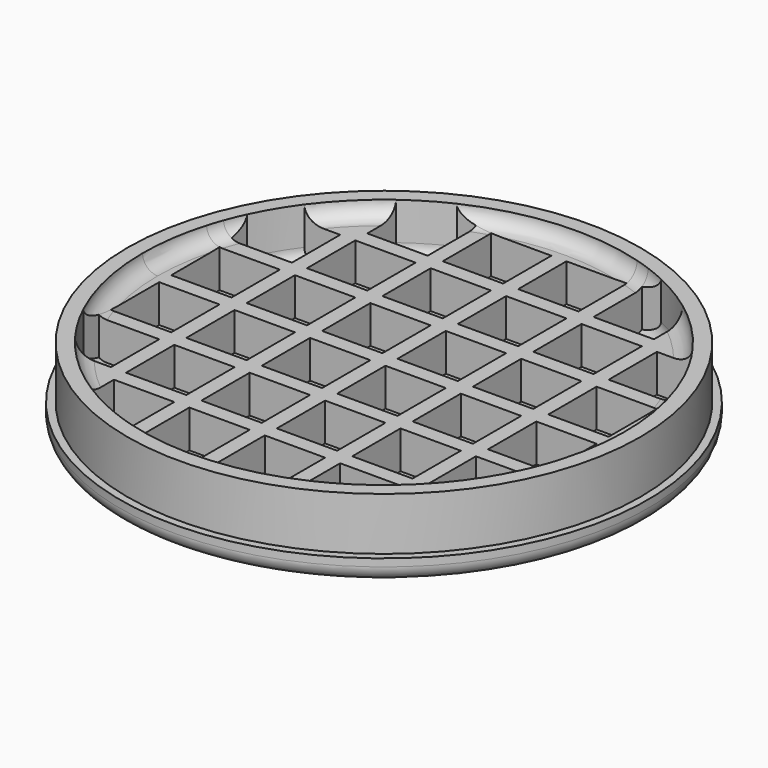
from build123d import *

# Parameters (mm, degrees)
F2_W          = 8
F2_H          = 8
F3_DEPTH      = 5
F4_T4_ANGLE   = 67.9228184519
F4_T10_ANGLE  = 67.9228184519
F4_T15_ANGLE  = 67.9228184519
F4_T21_ANGLE  = 35.0580450012
F4_T27_ANGLE  = 33.9605763761
F4_T33_ANGLE  = 33.9605763761
F4_T38_ANGLE  = 33.9605763761
F4_T43_ANGLE  = 33.9605763761
F4_T49_ANGLE  = 35.0580450012
F4_T55_ANGLE  = 67.9228184519
F4_T61_ANGLE  = 67.9228184519
F4_T66_ANGLE  = 67.9228184519
F4_T72_ANGLE  = 35.0580450012
F4_T78_ANGLE  = 67.9228184519
F4_T84_ANGLE  = 67.9228184519
F4_T89_ANGLE  = 67.9228184519
F4_T95_ANGLE  = 35.0580450012
F4_T101_ANGLE = 35.5875535678
F4_T106_ANGLE = 35.5875535678
F4_T111_ANGLE = 35.5875535678
F4_T116_ANGLE = 35.5875535678
F4_T121_ANGLE = 35.5875535678
F4_T126_ANGLE = 35.5875535678
F4_T131_ANGLE = 35.5875535678
F4_T136_ANGLE = 35.5875535678


# Not quite as in the source:
# - a fillet or chamfer that OpenCascade refuses, or shapes differently, is made with other operations: its cross-section is extruded or revolved along the edge and cut away or added


with BuildPart() as f1:
    # F0 (on Front) → F1 (revolve)
    with BuildSketch(Plane.XZ):
        with BuildLine():
            Line((-33, 0), (0, 0))
            Line((0, 0), (0, 3))
            Line((0, 3), (-32, 3))
            Line((-32, 3), (-32, 10))
            Line((-32, 10), (-34, 10))
            Line((-34, 10), (-34, 3))
            Line((-34, 3), (-35, 3))
            Line((-35, 3), (-35, 2))
            ThreePointArc((-35, 2), (-34.4142135624, 0.5857864376), (-33, 0))
        make_face()
    revolve(axis=Axis((0, 0, 1.5), (0, 0, -1)))

    # F2 (on face) → F3 (join)
    with BuildSketch(Plane.XY.offset(3)):
        with BuildLine():
            Line((11, 21), (11, 29))
            Line((11, 29), (13.5277492585, 29))
            ThreePointArc((13.5277492585, 29), (0, 32), (-13.5277492585, 29))
            Line((-13.5277492585, 29), (-11, 29))
            Line((-11, 29), (-11, 21))
            Line((-11, 21), (-19, 21))
            Line((-19, 21), (-19, 25.7487863792))
            ThreePointArc((-19, 25.7487863792), (-22.627416998, 22.627416998), (-25.7487863792, 19))
            Line((-25.7487863792, 19), (-21, 19))
            Line((-21, 19), (-21, 11))
            Line((-21, 11), (-29, 11))
            Line((-29, 11), (-29, 13.5277492585))
            ThreePointArc((-29, 13.5277492585), (-32, 0), (-29, -13.5277492585))
            Line((-29, -13.5277492585), (-29, -11))
            Line((-29, -11), (-21, -11))
            Line((-21, -11), (-21, -19))
            Line((-21, -19), (-25.7487863792, -19))
            ThreePointArc((-25.7487863792, -19), (-22.627416998, -22.627416998), (-19, -25.7487863792))
            Line((-19, -25.7487863792), (-19, -21))
            Line((-19, -21), (-11, -21))
            Line((-11, -21), (-11, -29))
            Line((-11, -29), (-13.5277492585, -29))
            ThreePointArc((-13.5277492585, -29), (0, -32), (13.5277492585, -29))
            Line((13.5277492585, -29), (11, -29))
            Line((11, -29), (11, -21))
            Line((11, -21), (19, -21))
            Line((19, -21), (19, -25.7487863792))
            ThreePointArc((19, -25.7487863792), (22.627416998, -22.627416998), (25.7487863792, -19))
            Line((25.7487863792, -19), (21, -19))
            Line((21, -19), (21, -11))
            Line((21, -11), (29, -11))
            Line((29, -11), (29, -13.5277492585))
            ThreePointArc((29, -13.5277492585), (32, 0), (29, 13.5277492585))
            Line((29, 13.5277492585), (29, 11))
            Line((29, 11), (21, 11))
            Line((21, 11), (21, 19))
            Line((21, 19), (25.7487863792, 19))
            ThreePointArc((25.7487863792, 19), (22.627416998, 22.627416998), (19, 25.7487863792))
            Line((19, 25.7487863792), (19, 21))
            Line((19, 21), (11, 21))
        make_face()
        with Locations((-5, -25)):
            Rectangle(F2_W, F2_H, mode=Mode.SUBTRACT)
        with Locations((-25, -5)):
            Rectangle(F2_W, F2_H, mode=Mode.SUBTRACT)
        with Locations((-15, -15)):
            Rectangle(F2_W, F2_H, mode=Mode.SUBTRACT)
        with Locations((-5, -15)):
            Rectangle(F2_W, F2_H, mode=Mode.SUBTRACT)
        with Locations((-15, -5)):
            Rectangle(F2_W, F2_H, mode=Mode.SUBTRACT)
        with Locations((-5, -5)):
            Rectangle(F2_W, F2_H, mode=Mode.SUBTRACT)
        with Locations((5, -25)):
            Rectangle(F2_W, F2_H, mode=Mode.SUBTRACT)
        with Locations((5, -15)):
            Rectangle(F2_W, F2_H, mode=Mode.SUBTRACT)
        with Locations((15, -15)):
            Rectangle(F2_W, F2_H, mode=Mode.SUBTRACT)
        with Locations((5, -5)):
            Rectangle(F2_W, F2_H, mode=Mode.SUBTRACT)
        with Locations((15, -5)):
            Rectangle(F2_W, F2_H, mode=Mode.SUBTRACT)
        with Locations((25, -5)):
            Rectangle(F2_W, F2_H, mode=Mode.SUBTRACT)
        with Locations((-25, 5)):
            Rectangle(F2_W, F2_H, mode=Mode.SUBTRACT)
        with Locations((-15, 5)):
            Rectangle(F2_W, F2_H, mode=Mode.SUBTRACT)
        with Locations((-5, 5)):
            Rectangle(F2_W, F2_H, mode=Mode.SUBTRACT)
        with Locations((-15, 15)):
            Rectangle(F2_W, F2_H, mode=Mode.SUBTRACT)
        with Locations((-5, 15)):
            Rectangle(F2_W, F2_H, mode=Mode.SUBTRACT)
        with Locations((-5, 25)):
            Rectangle(F2_W, F2_H, mode=Mode.SUBTRACT)
        with Locations((5, 5)):
            Rectangle(F2_W, F2_H, mode=Mode.SUBTRACT)
        with Locations((15, 5)):
            Rectangle(F2_W, F2_H, mode=Mode.SUBTRACT)
        with Locations((5, 15)):
            Rectangle(F2_W, F2_H, mode=Mode.SUBTRACT)
        with Locations((15, 15)):
            Rectangle(F2_W, F2_H, mode=Mode.SUBTRACT)
        with Locations((25, 5)):
            Rectangle(F2_W, F2_H, mode=Mode.SUBTRACT)
        with Locations((5, 25)):
            Rectangle(F2_W, F2_H, mode=Mode.SUBTRACT)
    extrude(amount=F3_DEPTH)

    # F4: fillet of radius 2 on 17 edges, made by hand


with BuildPart() as f4_tool2:
    # F4_s3 → F4_t4 (revolve)
    with BuildSketch(Plane(origin=(0, 0, 0), x_dir=(0, 0, 1), z_dir=(-0.8294140211, 0.55863439, 0))):
        with BuildLine():
            ThreePointArc((10, -32), (8.5857864376, -31.4142135624), (8, -30))
            Line((8, -30), (8, -32))
            Line((8, -32), (10, -32))
        make_face()
    revolve(axis=Axis((0, 0, 8), (0, 0, 1)), revolution_arc=F4_T4_ANGLE)

    split(bisect_by=Plane.YZ.offset(-11), keep=Keep.TOP)

    split(bisect_by=Plane.YZ.offset(-9), keep=Keep.BOTTOM)


with BuildPart() as f1_1:
    add(f1.part)

    # F4_t1: union F4_tool2
    add(f4_tool2.part)


with BuildPart() as f4_tool8:
    # F4_s9 → F4_t10 (revolve)
    with BuildSketch(Plane(origin=(0, 0, 0), x_dir=(0, 0, 1), z_dir=(-0.8294140211, 0.55863439, 0))):
        with BuildLine():
            ThreePointArc((10, -32), (8.5857864376, -31.4142135624), (8, -30))
            Line((8, -30), (8, -32))
            Line((8, -32), (10, -32))
        make_face()
    revolve(axis=Axis((0, 0, 8), (0, 0, 1)), revolution_arc=F4_T10_ANGLE)

    split(bisect_by=Plane.XZ.offset(29), keep=Keep.TOP)


with BuildPart() as f1_2:
    add(f1_1.part)

    # F4_t7: union F4_tool8
    add(f4_tool8.part)


with BuildPart() as f4_tool13:
    # F4_s14 → F4_t15 (revolve)
    with BuildSketch(Plane(origin=(0, 0, 0), x_dir=(0, 0, 1), z_dir=(-0.8294140211, 0.55863439, 0))):
        with BuildLine():
            ThreePointArc((10, -32), (8.5857864376, -31.4142135624), (8, -30))
            Line((8, -30), (8, -32))
            Line((8, -32), (10, -32))
        make_face()
    revolve(axis=Axis((0, 0, 8), (0, 0, 1)), revolution_arc=F4_T15_ANGLE)

    split(bisect_by=Plane.YZ.offset(11), keep=Keep.BOTTOM)

    split(bisect_by=Plane.YZ.offset(9), keep=Keep.TOP)


with BuildPart() as f1_3:
    add(f1_2.part)

    # F4_t12: union F4_tool13
    add(f4_tool13.part)


with BuildPart() as f4_tool19:
    # F4_s20 → F4_t21 (revolve)
    with BuildSketch(Plane(origin=(0, 0, 0), x_dir=(0, 0, 1), z_dir=(-0.4612992492, 0.8872446127, 0))):
        with BuildLine():
            ThreePointArc((10, -32), (8.5857864376, -31.4142135624), (8, -30))
            Line((8, -30), (8, -32))
            Line((8, -32), (10, -32))
        make_face()
    revolve(axis=Axis((0, 0, 8), (0, 0, 1)), revolution_arc=F4_T21_ANGLE)

    split(bisect_by=Plane.XZ.offset(19), keep=Keep.TOP)

    split(bisect_by=Plane.YZ.offset(-19), keep=Keep.BOTTOM)


with BuildPart() as f1_4:
    add(f1_3.part)

    # F4_t18: union F4_tool19
    add(f4_tool19.part)


with BuildPart() as f4_tool25:
    # F4_s26 → F4_t27 (revolve)
    with BuildSketch(Plane(origin=(0, 0, 0), x_dir=(0, 0, 1), z_dir=(0.5586223336, 0.8294221413, 0))):
        with BuildLine():
            ThreePointArc((10, -32), (8.5857864376, -31.4142135624), (8, -30))
            Line((8, -30), (8, -32))
            Line((8, -32), (10, -32))
        make_face()
    revolve(axis=Axis((0, 0, 8), (0, 0, 1)), revolution_arc=F4_T27_ANGLE)

    split(bisect_by=Plane.XZ.offset(-11), keep=Keep.TOP)

    split(bisect_by=Plane.XZ.offset(-9), keep=Keep.BOTTOM)


with BuildPart() as f1_5:
    add(f1_4.part)

    # F4_t24: union F4_tool25
    add(f4_tool25.part)


with BuildPart() as f4_tool31:
    # F4_s32 → F4_t33 (revolve)
    with BuildSketch(Plane(origin=(0, 0, 0), x_dir=(0, 0, 1), z_dir=(0.5586223336, 0.8294221413, 0))):
        with BuildLine():
            ThreePointArc((10, -32), (8.5857864376, -31.4142135624), (8, -30))
            Line((8, -30), (8, -32))
            Line((8, -32), (10, -32))
        make_face()
    revolve(axis=Axis((0, 0, 8), (0, 0, 1)), revolution_arc=F4_T33_ANGLE)

    split(bisect_by=Plane.YZ.offset(-29), keep=Keep.BOTTOM)


with BuildPart() as f1_6:
    add(f1_5.part)

    # F4_t30: union F4_tool31
    add(f4_tool31.part)


with BuildPart() as f4_tool36:
    # F4_s37 → F4_t38 (revolve)
    with BuildSketch(Plane.XZ):
        with BuildLine():
            ThreePointArc((-32, 10), (-31.4142135624, 8.5857864376), (-30, 8))
            Line((-30, 8), (-32, 8))
            Line((-32, 8), (-32, 10))
        make_face()
    revolve(axis=Axis((0, 0, 8), (0, 0, 1)), revolution_arc=F4_T38_ANGLE)

    split(bisect_by=Plane.YZ.offset(-29), keep=Keep.BOTTOM)


with BuildPart() as f1_7:
    add(f1_6.part)

    # F4_t35: union F4_tool36
    add(f4_tool36.part)


with BuildPart() as f4_tool41:
    # F4_s42 → F4_t43 (revolve)
    with BuildSketch(Plane.XZ):
        with BuildLine():
            ThreePointArc((-32, 10), (-31.4142135624, 8.5857864376), (-30, 8))
            Line((-30, 8), (-32, 8))
            Line((-32, 8), (-32, 10))
        make_face()
    revolve(axis=Axis((0, 0, 8), (0, 0, 1)), revolution_arc=F4_T43_ANGLE)

    split(bisect_by=Plane.XZ.offset(11), keep=Keep.BOTTOM)

    split(bisect_by=Plane.XZ.offset(9), keep=Keep.TOP)


with BuildPart() as f1_8:
    add(f1_7.part)

    # F4_t40: union F4_tool41
    add(f4_tool41.part)


with BuildPart() as f4_tool47:
    # F4_s48 → F4_t49 (revolve)
    with BuildSketch(Plane(origin=(0, 0, 0), x_dir=(0, 0, 1), z_dir=(-0.8872446127, -0.4612992492, 0))):
        with BuildLine():
            ThreePointArc((10, -32), (8.5857864376, -31.4142135624), (8, -30))
            Line((8, -30), (8, -32))
            Line((8, -32), (10, -32))
        make_face()
    revolve(axis=Axis((0, 0, 8), (0, 0, 1)), revolution_arc=F4_T49_ANGLE)

    split(bisect_by=Plane.YZ.offset(19), keep=Keep.TOP)

    split(bisect_by=Plane.XZ.offset(19), keep=Keep.TOP)


with BuildPart() as f1_9:
    add(f1_8.part)

    # F4_t46: union F4_tool47
    add(f4_tool47.part)


with BuildPart() as f4_tool53:
    # F4_s54 → F4_t55 (revolve)
    with BuildSketch(Plane(origin=(0, 0, 0), x_dir=(0, 0, 1), z_dir=(-0.55863439, -0.8294140211, 0))):
        with BuildLine():
            ThreePointArc((10, -32), (8.5857864376, -31.4142135624), (8, -30))
            Line((8, -30), (8, -32))
            Line((8, -32), (10, -32))
        make_face()
    revolve(axis=Axis((0, 0, 8), (0, 0, 1)), revolution_arc=F4_T55_ANGLE)

    split(bisect_by=Plane.XZ.offset(11), keep=Keep.BOTTOM)

    split(bisect_by=Plane.XZ.offset(9), keep=Keep.TOP)


with BuildPart() as f1_10:
    add(f1_9.part)

    # F4_t52: union F4_tool53
    add(f4_tool53.part)


with BuildPart() as f4_tool59:
    # F4_s60 → F4_t61 (revolve)
    with BuildSketch(Plane(origin=(0, 0, 0), x_dir=(0, 0, 1), z_dir=(-0.55863439, -0.8294140211, 0))):
        with BuildLine():
            ThreePointArc((10, -32), (8.5857864376, -31.4142135624), (8, -30))
            Line((8, -30), (8, -32))
            Line((8, -32), (10, -32))
        make_face()
    revolve(axis=Axis((0, 0, 8), (0, 0, 1)), revolution_arc=F4_T61_ANGLE)

    split(bisect_by=Plane.YZ.offset(29), keep=Keep.TOP)


with BuildPart() as f1_11:
    add(f1_10.part)

    # F4_t58: union F4_tool59
    add(f4_tool59.part)


with BuildPart() as f4_tool64:
    # F4_s65 → F4_t66 (revolve)
    with BuildSketch(Plane(origin=(0, 0, 0), x_dir=(0, 0, 1), z_dir=(-0.55863439, -0.8294140211, 0))):
        with BuildLine():
            ThreePointArc((10, -32), (8.5857864376, -31.4142135624), (8, -30))
            Line((8, -30), (8, -32))
            Line((8, -32), (10, -32))
        make_face()
    revolve(axis=Axis((0, 0, 8), (0, 0, 1)), revolution_arc=F4_T66_ANGLE)

    split(bisect_by=Plane.XZ.offset(-11), keep=Keep.TOP)

    split(bisect_by=Plane.XZ.offset(-9), keep=Keep.BOTTOM)


with BuildPart() as f1_12:
    add(f1_11.part)

    # F4_t63: union F4_tool64
    add(f4_tool64.part)


with BuildPart() as f4_tool70:
    # F4_s71 → F4_t72 (revolve)
    with BuildSketch(Plane(origin=(0, 0, 0), x_dir=(0, 0, 1), z_dir=(0.4612992492, -0.8872446127, 0))):
        with BuildLine():
            ThreePointArc((10, -32), (8.5857864376, -31.4142135624), (8, -30))
            Line((8, -30), (8, -32))
            Line((8, -32), (10, -32))
        make_face()
    revolve(axis=Axis((0, 0, 8), (0, 0, 1)), revolution_arc=F4_T72_ANGLE)

    split(bisect_by=Plane.XZ.offset(-19), keep=Keep.BOTTOM)

    split(bisect_by=Plane.YZ.offset(19), keep=Keep.TOP)


with BuildPart() as f1_13:
    add(f1_12.part)

    # F4_t69: union F4_tool70
    add(f4_tool70.part)


with BuildPart() as f4_tool76:
    # F4_s77 → F4_t78 (revolve)
    with BuildSketch(Plane(origin=(0, 0, 0), x_dir=(0, 0, 1), z_dir=(0.8294140211, -0.55863439, 0))):
        with BuildLine():
            ThreePointArc((10, -32), (8.5857864376, -31.4142135624), (8, -30))
            Line((8, -30), (8, -32))
            Line((8, -32), (10, -32))
        make_face()
    revolve(axis=Axis((0, 0, 8), (0, 0, 1)), revolution_arc=F4_T78_ANGLE)

    split(bisect_by=Plane.YZ.offset(11), keep=Keep.BOTTOM)

    split(bisect_by=Plane.YZ.offset(9), keep=Keep.TOP)


with BuildPart() as f1_14:
    add(f1_13.part)

    # F4_t75: union F4_tool76
    add(f4_tool76.part)


with BuildPart() as f4_tool82:
    # F4_s83 → F4_t84 (revolve)
    with BuildSketch(Plane(origin=(0, 0, 0), x_dir=(0, 0, 1), z_dir=(0.8294140211, -0.55863439, 0))):
        with BuildLine():
            ThreePointArc((10, -32), (8.5857864376, -31.4142135624), (8, -30))
            Line((8, -30), (8, -32))
            Line((8, -32), (10, -32))
        make_face()
    revolve(axis=Axis((0, 0, 8), (0, 0, 1)), revolution_arc=F4_T84_ANGLE)

    split(bisect_by=Plane.XZ.offset(-29), keep=Keep.BOTTOM)


with BuildPart() as f1_15:
    add(f1_14.part)

    # F4_t81: union F4_tool82
    add(f4_tool82.part)


with BuildPart() as f4_tool87:
    # F4_s88 → F4_t89 (revolve)
    with BuildSketch(Plane(origin=(0, 0, 0), x_dir=(0, 0, 1), z_dir=(0.8294140211, -0.55863439, 0))):
        with BuildLine():
            ThreePointArc((10, -32), (8.5857864376, -31.4142135624), (8, -30))
            Line((8, -30), (8, -32))
            Line((8, -32), (10, -32))
        make_face()
    revolve(axis=Axis((0, 0, 8), (0, 0, 1)), revolution_arc=F4_T89_ANGLE)

    split(bisect_by=Plane.YZ.offset(-11), keep=Keep.TOP)

    split(bisect_by=Plane.YZ.offset(-9), keep=Keep.BOTTOM)


with BuildPart() as f1_16:
    add(f1_15.part)

    # F4_t86: union F4_tool87
    add(f4_tool87.part)


with BuildPart() as f4_tool93:
    # F4_s94 → F4_t95 (revolve)
    with BuildSketch(Plane(origin=(0, 0, 0), x_dir=(0, 0, 1), z_dir=(0.8872446127, 0.4612992492, 0))):
        with BuildLine():
            ThreePointArc((10, -32), (8.5857864376, -31.4142135624), (8, -30))
            Line((8, -30), (8, -32))
            Line((8, -32), (10, -32))
        make_face()
    revolve(axis=Axis((0, 0, 8), (0, 0, 1)), revolution_arc=F4_T95_ANGLE)

    split(bisect_by=Plane.YZ.offset(-19), keep=Keep.BOTTOM)

    split(bisect_by=Plane.XZ.offset(-19), keep=Keep.BOTTOM)


with BuildPart() as f1_17:
    add(f1_16.part)

    # F4_t92: union F4_tool93
    add(f4_tool93.part)


with BuildPart() as f4_tool99:
    # F4_s100 → F4_t101 (revolve)
    with BuildSketch(Plane(origin=(0, 0, 0), x_dir=(0, 0, 1), z_dir=(-0.7024500388, -0.711733056, 0))):
        with BuildLine():
            ThreePointArc((5, 32), (3.5857864376, 31.4142135624), (3, 30))
            Line((3, 30), (3, 32))
            Line((3, 32), (5, 32))
        make_face()
    revolve(axis=Axis((0, 0, 3), (0, 0, -1)), revolution_arc=F4_T101_ANGLE)

    split(bisect_by=Plane.YZ.offset(-9), keep=Keep.BOTTOM)


with BuildPart() as f1_18:
    add(f1_17.part)

    # F4_t98: union F4_tool99
    add(f4_tool99.part)


with BuildPart() as f4_tool104:
    # F4_s105 → F4_t106 (revolve)
    with BuildSketch(Plane(origin=(0, 0, 0), x_dir=(0, 0, 1), z_dir=(-0.1700124593, -0.9854419129, 0))):
        with BuildLine():
            ThreePointArc((5, 32), (3.5857864376, 31.4142135624), (3, 30))
            Line((3, 30), (3, 32))
            Line((3, 32), (5, 32))
        make_face()
    revolve(axis=Axis((0, 0, 3), (0, 0, -1)), revolution_arc=F4_T106_ANGLE)

    split(bisect_by=Plane.XZ.offset(-9), keep=Keep.BOTTOM)


with BuildPart() as f1_19:
    add(f1_18.part)

    # F4_t103: union F4_tool104
    add(f4_tool104.part)


with BuildPart() as f4_tool109:
    # F4_s110 → F4_t111 (revolve)
    with BuildSketch(Plane(origin=(0, 0, 0), x_dir=(0, 0, 1), z_dir=(-0.9854419129, 0.1700124593, 0))):
        with BuildLine():
            ThreePointArc((5, 32), (3.5857864376, 31.4142135624), (3, 30))
            Line((3, 30), (3, 32))
            Line((3, 32), (5, 32))
        make_face()
    revolve(axis=Axis((0, 0, 3), (0, 0, -1)), revolution_arc=F4_T111_ANGLE)

    split(bisect_by=Plane.YZ.offset(9), keep=Keep.TOP)


with BuildPart() as f1_20:
    add(f1_19.part)

    # F4_t108: union F4_tool109
    add(f4_tool109.part)


with BuildPart() as f4_tool114:
    # F4_s115 → F4_t116 (revolve)
    with BuildSketch(Plane(origin=(0, 0, 0), x_dir=(0, 0, 1), z_dir=(0.711733056, -0.7024500388, 0))):
        with BuildLine():
            ThreePointArc((5, 32), (3.5857864376, 31.4142135624), (3, 30))
            Line((3, 30), (3, 32))
            Line((3, 32), (5, 32))
        make_face()
    revolve(axis=Axis((0, 0, 3), (0, 0, -1)), revolution_arc=F4_T116_ANGLE)

    split(bisect_by=Plane.XZ.offset(9), keep=Keep.TOP)


with BuildPart() as f1_21:
    add(f1_20.part)

    # F4_t113: union F4_tool114
    add(f4_tool114.part)


with BuildPart() as f4_tool119:
    # F4_s120 → F4_t121 (revolve)
    with BuildSketch(Plane(origin=(0, 0, 0), x_dir=(0, 0, 1), z_dir=(0.9854419129, -0.1700124593, 0))):
        with BuildLine():
            ThreePointArc((5, 32), (3.5857864376, 31.4142135624), (3, 30))
            Line((3, 30), (3, 32))
            Line((3, 32), (5, 32))
        make_face()
    revolve(axis=Axis((0, 0, 3), (0, 0, -1)), revolution_arc=F4_T121_ANGLE)

    split(bisect_by=Plane.YZ.offset(-9), keep=Keep.BOTTOM)


with BuildPart() as f1_22:
    add(f1_21.part)

    # F4_t118: union F4_tool119
    add(f4_tool119.part)


with BuildPart() as f4_tool124:
    # F4_s125 → F4_t126 (revolve)
    with BuildSketch(Plane(origin=(0, 0, 0), x_dir=(0, 0, 1), z_dir=(0.7024500388, 0.711733056, 0))):
        with BuildLine():
            ThreePointArc((5, 32), (3.5857864376, 31.4142135624), (3, 30))
            Line((3, 30), (3, 32))
            Line((3, 32), (5, 32))
        make_face()
    revolve(axis=Axis((0, 0, 3), (0, 0, -1)), revolution_arc=F4_T126_ANGLE)

    split(bisect_by=Plane.YZ.offset(9), keep=Keep.TOP)


with BuildPart() as f1_23:
    add(f1_22.part)

    # F4_t123: union F4_tool124
    add(f4_tool124.part)


with BuildPart() as f4_tool129:
    # F4_s130 → F4_t131 (revolve)
    with BuildSketch(Plane(origin=(0, 0, 0), x_dir=(0, 0, 1), z_dir=(0.1700124593, 0.9854419129, 0))):
        with BuildLine():
            ThreePointArc((5, 32), (3.5857864376, 31.4142135624), (3, 30))
            Line((3, 30), (3, 32))
            Line((3, 32), (5, 32))
        make_face()
    revolve(axis=Axis((0, 0, 3), (0, 0, -1)), revolution_arc=F4_T131_ANGLE)

    split(bisect_by=Plane.XZ.offset(9), keep=Keep.TOP)


with BuildPart() as f1_24:
    add(f1_23.part)

    # F4_t128: union F4_tool129
    add(f4_tool129.part)


with BuildPart() as f4_tool134:
    # F4_s135 → F4_t136 (revolve)
    with BuildSketch(Plane(origin=(0, 0, 0), x_dir=(0, 0, 1), z_dir=(-0.711733056, 0.7024500388, 0))):
        with BuildLine():
            ThreePointArc((5, 32), (3.5857864376, 31.4142135624), (3, 30))
            Line((3, 30), (3, 32))
            Line((3, 32), (5, 32))
        make_face()
    revolve(axis=Axis((0, 0, 3), (0, 0, -1)), revolution_arc=F4_T136_ANGLE)

    split(bisect_by=Plane.XZ.offset(-9), keep=Keep.BOTTOM)


with BuildPart() as f1_25:
    add(f1_24.part)

    # F4_t133: union F4_tool134
    add(f4_tool134.part)


solid = f1_25.part
